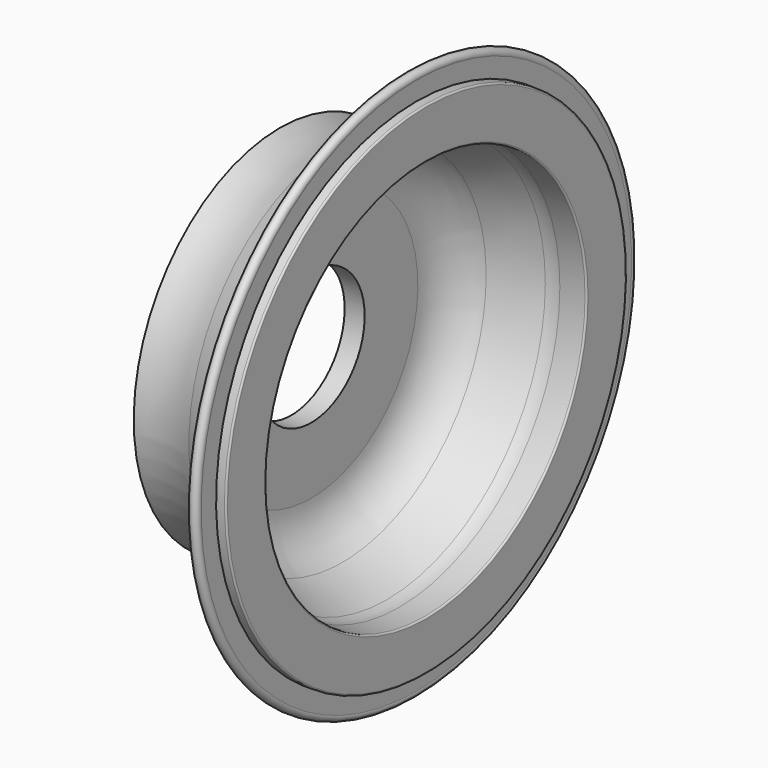
from build123d import *

# Parameters (mm, degrees)
F2_R = 0.5


# Not quite as in the source:
# - a feature names something its author has since deleted; it is built from what else it names


with BuildPart() as f1:
    # F0 (on Front) → F1 (revolve)
    with BuildSketch(Plane.XZ):
        with BuildLine():
            Line((37.5, 60), (37.5, 75))
            Line((37.5, 75), (34.5, 75))
            Line((34.5, 75), (34.5, 80.5609297038))
            ThreePointArc((34.5, 80.5609297038), (33.2876789928, 82.4834841439), (31.5656997263, 81))
            Line((31.5656997263, 81), (31.5656997263, 71.2215793345))
            ThreePointArc((31.5656997263, 71.2215793345), (29.8659918821, 65.6443802051), (25.3446697006, 61.9631028976))
            Line((25.3446697006, 61.9631028976), (11.3369099228, 56.245649927))
            ThreePointArc((11.3369099228, 56.245649927), (2.5887477284, 54.1329815199), (-6.3923836679, 54.7100330088))
            ThreePointArc((-6.3923836679, 54.7100330088), (-3.8589680114, 47.5076038142), (-3, 39.9210792379))
            Line((-3, 39.9210792379), (-3, 20))
            Line((-3, 20), (0, 20))
            Line((0, 20), (3, 20))
            Line((3, 20), (3, 39.9210792379))
            ThreePointArc((3, 39.9210792379), (5.5495617663, 48.2868779319), (12.3315450386, 53.8087938933))
            Line((12.3315450386, 53.8087938933), (25.6832672705, 59.258476437))
            ThreePointArc((25.6832672705, 59.258476437), (27.5367197, 59.8128681936), (29.4622372448, 60))
            Line((29.4622372448, 60), (37.5, 60))
        make_face()
    revolve(axis=Axis((8.4361489862, 0, 0), (1, 0, 0)))

    # F2
    f2_edges = [f1.edges().sort_by_distance(p)[0] for p in [
        (37.5, 0, -60),
        (37.5, 0, -75),
    ]]
    fillet(f2_edges, radius=F2_R)


solid = f1.part
